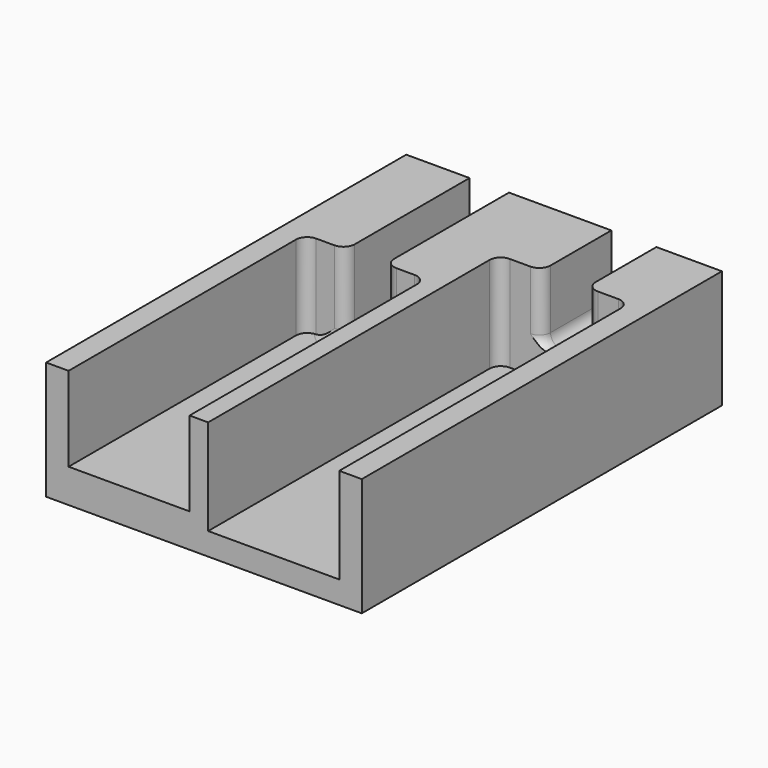
from build123d import *

# Parameters (mm, degrees)
F0_W         = 3.5
F0_H         = 13.75
F0_W_2       = 4
F0_H_2       = 7.75
F1_DEPTH     = 2
F2_DEPTH     = 8.5
F3_DEPTH     = 1
F4_DEPTH     = 2.25
F5_R         = 1
F6_T1_DEPTH  = 12.75
F6_T3_DEPTH  = 6.75
F6_T6_ANGLE  = 233.2969892374
F6_T8_ANGLE  = 233.2969892374
F6_T12_ANGLE = 233.2969892374
F6_T17_ANGLE = 233.2969892374


# Not quite as in the source:
# - a fillet or chamfer that OpenCascade refuses, or shapes differently, is made with other operations: its cross-section is extruded or revolved along the edge and cut away or added


with BuildPart() as f1:
    # F0 (on Top) → F1 (new body)
    with BuildSketch(Plane.XY):
        Polygon((-12.025, -20), (-1.275, -20), (-1.275, 6.25), (-4.9, 6.25), (-8.4, 6.25), (-12.025, 6.25), align=None)
        Polygon((-14.025, -20), (-12.025, -20), (-12.025, 6.25), (-8.4, 6.25), (-8.4, 20), (-14.025, 20), align=None)
        Polygon((-1.275, -20), (0.375, -20), (0.375, 12.25), (4.2, 12.25), (4.2, 20), (-4.9, 20), (-4.9, 6.25), (-1.275, 6.25), align=None)
        with Locations((-6.65, 13.125)):
            Rectangle(F0_W, F0_H)
        with Locations((6.2, 16.125)):
            Rectangle(F0_W_2, F0_H_2)
        Polygon((0.375, -20), (12.025, -20), (12.025, 12.25), (8.2, 12.25), (4.2, 12.25), (0.375, 12.25), align=None)
        Polygon((12.025, -20), (14.025, -20), (14.025, 20), (8.2, 20), (8.2, 12.25), (12.025, 12.25), align=None)
    extrude(amount=-F1_DEPTH)

    # F0 (on Top) → F2 (join)
    with BuildSketch(Plane.XY):
        Polygon((-14.025, -20), (-12.025, -20), (-12.025, 6.25), (-8.4, 6.25), (-8.4, 20), (-14.025, 20), align=None)
        Polygon((-1.275, -20), (0.375, -20), (0.375, 12.25), (4.2, 12.25), (4.2, 20), (-4.9, 20), (-4.9, 6.25), (-1.275, 6.25), align=None)
        Polygon((12.025, -20), (14.025, -20), (14.025, 20), (8.2, 20), (8.2, 12.25), (12.025, 12.25), align=None)
    extrude(amount=F2_DEPTH)

    # F0 (on Top) → F3 (join)
    with BuildSketch(Plane.XY):
        Polygon((-12.025, -20), (-1.275, -20), (-1.275, 6.25), (-4.9, 6.25), (-8.4, 6.25), (-12.025, 6.25), align=None)
        with Locations((-6.65, 13.125)):
            Rectangle(F0_W, F0_H)
    extrude(amount=F3_DEPTH)

    # F0 (on Top) → F4 (join)
    with BuildSketch(Plane.XY):
        with Locations((6.2, 16.125)):
            Rectangle(F0_W_2, F0_H_2)
    extrude(amount=F4_DEPTH)

    # F5
    f5_edges = [f1.edges().sort_by_distance(p)[0] for p in [
        (-12.025, 6.25, 4.75),
        (-8.4, 6.25, 4.75),
        (-4.9, 6.25, 4.75),
        (-1.275, 6.25, 4.75),
        (4.2, 12.25, 5.375),
        (8.2, 12.25, 5.375),
        (0.375, 12.25, 4.25),
        (12.025, 12.25, 4.25),
    ]]
    fillet(f5_edges, radius=F5_R)

    # F6: fillet of radius 1 on 8 edges, made by hand

    # F6_s2 → F6_t1 (join)
    with BuildSketch(Plane.XZ.offset(-20)):
        with BuildLine():
            ThreePointArc((-8.4, 2), (-8.1071067812, 1.2928932188), (-7.4, 1))
            Line((-7.4, 1), (-8.4, 1))
            Line((-8.4, 1), (-8.4, 2))
        make_face()
        with BuildLine():
            ThreePointArc((-5.9, 1), (-5.1928932188, 1.2928932188), (-4.9, 2))
            Line((-4.9, 2), (-4.9, 1))
            Line((-4.9, 1), (-5.9, 1))
        make_face()
    extrude(amount=F6_T1_DEPTH)

    # F6_s4 → F6_t3 (join)
    with BuildSketch(Plane.XZ.offset(-20)):
        with BuildLine():
            ThreePointArc((5.2, 2.25), (4.4928932188, 2.5428932188), (4.2, 3.25))
            Line((4.2, 3.25), (4.2, 2.25))
            Line((4.2, 2.25), (5.2, 2.25))
        make_face()
        with BuildLine():
            ThreePointArc((8.2, 3.25), (7.9071067812, 2.5428932188), (7.2, 2.25))
            Line((7.2, 2.25), (8.2, 2.25))
            Line((8.2, 2.25), (8.2, 3.25))
        make_face()
    extrude(amount=F6_T3_DEPTH)

    # F6_s5 → F6_t6 (revolve)
    with BuildSketch(Plane(origin=(-2.5682338051, -1.9145124235, 0), x_dir=(0, 0, 1), z_dir=(0.8017442393, 0.5976672776, 0))):
        with BuildLine():
            ThreePointArc((1, -13.4307181447), (1.2928932188, -12.7236113635), (2, -12.4307181447))
            Line((2, -12.4307181447), (1, -12.4307181447))
            Line((1, -12.4307181447), (1, -13.4307181447))
        make_face()
    revolve(axis=Axis((-9.4, 7.25, 1), (0, 0, 1)), revolution_arc=F6_T6_ANGLE)

    # F6_s7 → F6_t8 (revolve)
    with BuildSketch(Plane(origin=(-5.9809240707, 4.4585323247, 0), x_dir=(0, 0, 1), z_dir=(-0.8017442393, 0.5976672776, 0))):
        with BuildLine():
            ThreePointArc((1, 5.4817433521), (1.2928932188, 4.774636571), (2, 4.4817433521))
            Line((2, 4.4817433521), (1, 4.4817433521))
            Line((1, 4.4817433521), (1, 5.4817433521))
        make_face()
    revolve(axis=Axis((-3.9, 7.25, 1), (0, 0, -1)), revolution_arc=F6_T8_ANGLE)


with BuildPart() as f6_tool10:
    # F6_s11 → F6_t12 (revolve)
    with BuildSketch(Plane(origin=(8.4060261742, 6.2663459654, 0), x_dir=(0, 0, 1), z_dir=(0.8017442393, 0.5976672776, 0))):
        with BuildLine():
            ThreePointArc((2.25, -10.7105758823), (2.5428932188, -10.0034691011), (3.25, -9.7105758823))
            Line((3.25, -9.7105758823), (2.25, -9.7105758823))
            Line((2.25, -9.7105758823), (2.25, -10.7105758823))
        make_face()
    revolve(axis=Axis((3.2, 13.25, 2.25), (0, 0, 1)), revolution_arc=F6_T12_ANGLE)

    split(bisect_by=Plane.XZ.offset(-12.25), keep=Keep.BOTTOM)


with BuildPart() as f1_1:
    add(f1.part)

    # F6_t9: union F6_tool10
    add(f6_tool10.part)


with BuildPart() as f6_tool15:
    # F6_s16 → F6_t17 (revolve)
    with BuildSketch(Plane(origin=(-0.4353827411, 0.3245598844, 0), x_dir=(0, 0, 1), z_dir=(-0.8017442393, 0.5976672776, 0))):
        with BuildLine():
            ThreePointArc((3.25, 17.1216501249), (2.5428932188, 17.4145433437), (2.25, 18.1216501249))
            Line((2.25, 18.1216501249), (2.25, 17.1216501249))
            Line((2.25, 17.1216501249), (3.25, 17.1216501249))
        make_face()
    revolve(axis=Axis((9.2, 13.25, 2.25), (0, 0, -1)), revolution_arc=F6_T17_ANGLE)

    split(bisect_by=Plane.XZ.offset(-12.25), keep=Keep.BOTTOM)


with BuildPart() as f1_2:
    add(f1_1.part)

    # F6_t14: union F6_tool15
    add(f6_tool15.part)


solid = f1_2.part
